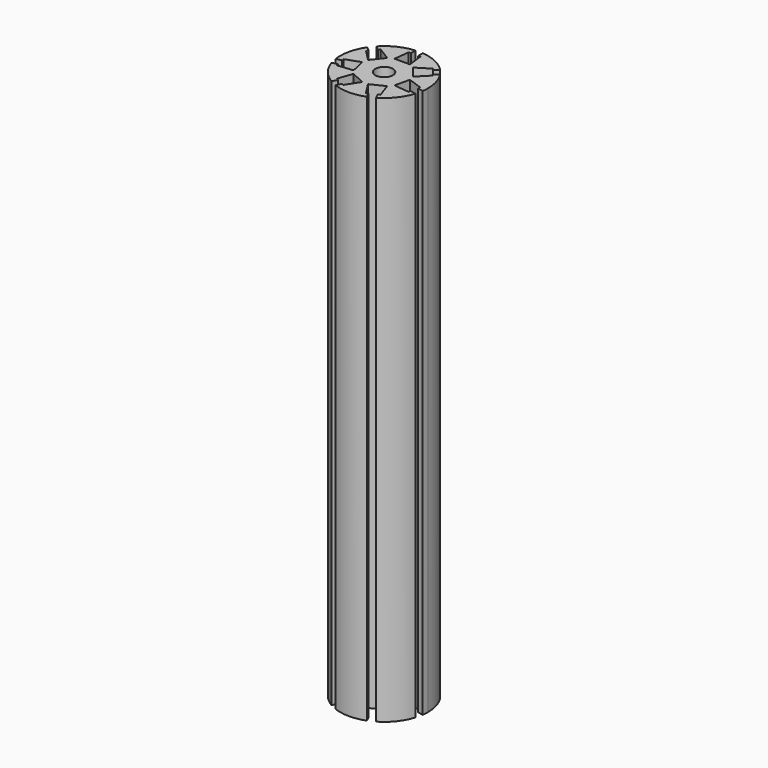
from build123d import *

# Parameters (mm, degrees)
F0_R     = 2.4
F1_DEPTH = 150


# Not quite as in the source:
# - a feature names something its author has since deleted; it is built from what else it names


with BuildPart() as f1:
    # F0 (on Top) → F1 (new body)
    with BuildSketch(Plane.XY):
        with BuildLine():
            ThreePointArc((11.8809631136, -1.6860354369), (11.9702037861, -0.8451161569), (12, 0))
            ThreePointArc((12, 0), (11.4820297491, 3.4875482565), (9.9728345264, 6.6740221388))
            Line((9.9728345264, 6.6740221388), (8.7545372195, 5.7024624569))
            Line((8.7545372195, 5.7024624569), (9.1286311006, 5.2333635674))
            Line((9.1286311006, 5.2333635674), (6.1566837752, 2.2237906583))
            Line((6.1566837752, 2.2237906583), (3.5380266074, 5.5074828847))
            Line((3.5380266074, 5.5074828847), (7.1334637347, 7.7352243113))
            Line((7.1334637347, 7.7352243113), (7.5075576158, 7.2661254218))
            Line((7.5075576158, 7.2661254218), (8.7258549227, 8.2376851038))
            ThreePointArc((8.7258549227, 8.2376851038), (5.2066048694, 10.8116264148), (1, 11.9582607431))
            Line((1, 11.9582607431), (1, 10.4))
            Line((1, 10.4), (1.6, 10.4))
            Line((1.6, 10.4), (2.1, 6.2))
            Line((2.1, 6.2), (-2.1, 6.2))
            Line((-2.1, 6.2), (-1.6, 10.4))
            Line((-1.6, 10.4), (-1, 10.4))
            Line((-1, 10.4), (-1, 11.9582607431))
            ThreePointArc((-1, 11.9582607431), (-5.2066048694, 10.8116264148), (-8.7258549227, 8.2376851038))
            Line((-8.7258549227, 8.2376851038), (-7.5075576158, 7.2661254218))
            Line((-7.5075576158, 7.2661254218), (-7.1334637347, 7.7352243113))
            Line((-7.1334637347, 7.7352243113), (-3.5380266074, 5.5074828847))
            Line((-3.5380266074, 5.5074828847), (-6.1566837752, 2.2237906583))
            Line((-6.1566837752, 2.2237906583), (-9.1286311006, 5.2333635674))
            Line((-9.1286311006, 5.2333635674), (-8.7545372195, 5.7024624569))
            Line((-8.7545372195, 5.7024624569), (-9.9728345264, 6.6740221388))
            ThreePointArc((-9.9728345264, 6.6740221388), (-11.6991349462, 2.6702512075), (-11.8809631136, -1.6860354369))
            Line((-11.8809631136, -1.6860354369), (-10.3617712206, -1.339289801))
            Line((-10.3617712206, -1.339289801), (-10.495283781, -0.7543330537))
            Line((-10.495283781, -0.7543330537), (-6.5118470168, 0.6677188251))
            Line((-6.5118470168, 0.6677188251), (-5.5772590942, -3.4269784061))
            Line((-5.5772590942, -3.4269784061), (-9.7832167924, -3.8741023726))
            Line((-9.7832167924, -3.8741023726), (-9.9167293527, -3.2891456253))
            Line((-9.9167293527, -3.2891456253), (-11.4359212456, -3.6358912612))
            ThreePointArc((-11.4359212456, -3.6358912612), (-9.3819777896, -7.4818776223), (-6.0894637525, -10.3401369047))
            Line((-6.0894637525, -10.3401369047), (-5.4133597547, -8.9361924871))
            Line((-5.4133597547, -8.9361924871), (-5.9539410755, -8.6758622436))
            Line((-5.9539410755, -8.6758622436), (-4.5821138051, -4.6748511288))
            Line((-4.5821138051, -4.6748511288), (-0.7980445599, -6.4971628331))
            Line((-0.7980445599, -6.4971628331), (-3.0708406982, -10.0642902088))
            Line((-3.0708406982, -10.0642902088), (-3.6114220189, -9.8039599653))
            Line((-3.6114220189, -9.8039599653), (-4.2875260167, -11.2079043829))
            ThreePointArc((-4.2875260167, -11.2079043829), (0, -12), (4.2875260167, -11.2079043829))
            Line((4.2875260167, -11.2079043829), (3.6114220189, -9.8039599653))
            Line((3.6114220189, -9.8039599653), (3.0708406982, -10.0642902088))
            Line((3.0708406982, -10.0642902088), (0.7980445599, -6.4971628331))
            Line((0.7980445599, -6.4971628331), (4.5821138051, -4.6748511288))
            Line((4.5821138051, -4.6748511288), (5.9539410755, -8.6758622436))
            Line((5.9539410755, -8.6758622436), (5.4133597547, -8.9361924871))
            Line((5.4133597547, -8.9361924871), (6.0894637525, -10.3401369047))
            ThreePointArc((6.0894637525, -10.3401369047), (9.3819777896, -7.4818776223), (11.4359212456, -3.6358912612))
            Line((11.4359212456, -3.6358912612), (9.9167293527, -3.2891456253))
            Line((9.9167293527, -3.2891456253), (9.7832167924, -3.8741023726))
            Line((9.7832167924, -3.8741023726), (5.5772590942, -3.4269784061))
            Line((5.5772590942, -3.4269784061), (6.5118470168, 0.6677188251))
            Line((6.5118470168, 0.6677188251), (10.495283781, -0.7543330537))
            Line((10.495283781, -0.7543330537), (10.3617712206, -1.339289801))
            Line((10.3617712206, -1.339289801), (11.8809631136, -1.6860354369))
        make_face()
        Circle(F0_R, mode=Mode.SUBTRACT)
    extrude(amount=F1_DEPTH)


solid = f1.part
